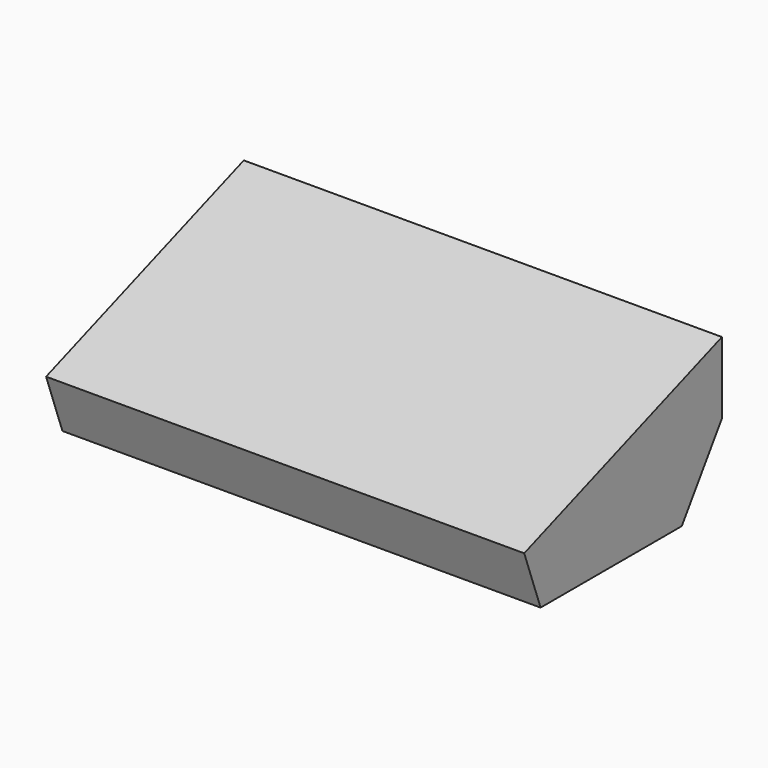
from build123d import *

# Parameters (mm, degrees)
F1_DEPTH = 400


# Not quite as in the source:
# - a feature names something its author has since deleted; it is built from what else it names


with BuildPart() as f1:
    # F0 (on Right) → F1 (new body)
    with BuildSketch(Plane.YZ):
        Polygon((140.2298494464, 75.2444315316), (-66.5025271265, 0), (-49.4015199602, -46.9846310393), (98.2558167472, -46.9846310393), (140.2298494464, 15.2444315316), align=None)
    extrude(amount=F1_DEPTH)


solid = f1.part
